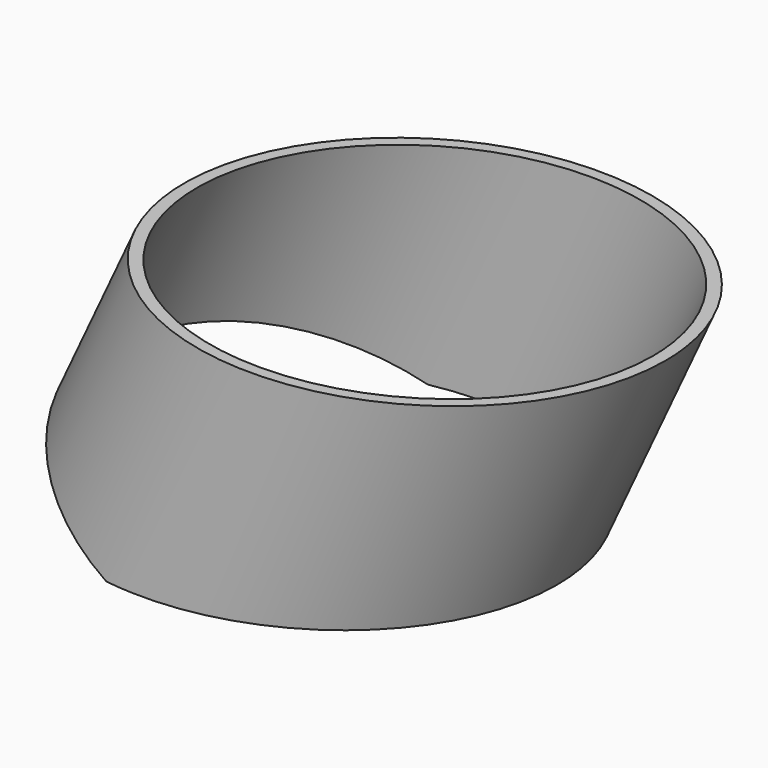
from build123d import *
from build123d import SkipClean  # not in build123d's __all__

# Parameters (mm, degrees)
F2_W     = 200
F2_H     = 100
F2_H_2   = 20
F3_DEPTH = 100
F2_W_2   = 75
F2_H_3   = 25
F6_DEPTH = 35
F8_W     = 96.0638802499
F8_H     = 5.2582259355
F9_DEPTH = 50


# Not quite as in the source:
# - ends of sketch curves that miss each other by under 0.0002 mm in the source are joined
# - a feature of the source that left no trace in its solid (it failed there, or was rolled back) is left out
# - a feature names something its author has since deleted; it is built from what else it names


with BuildPart() as f1:
    # F0 (on Front) → F1 (revolve)
    with BuildSketch(Plane.XZ):
        with BuildLine():
            add(Edge.make_bspline(
                [(45.9368361786, 26.8256458213), (91.5796084466, 124.7068868213), (26.32544778, 155.1354016666)],
                knots=[4.7123889804, 4.7123889804, 4.7123889804, 6.2831853072, 6.2831853072, 6.2831853072], degree=2, weights=[1, 0.7071067812, 1]))
            Line((26.32544778, 155.1354016666), (25.4802112565, 153.3227860925))
            add(Edge.make_bspline(
                [(44.1242206045, 27.6708823448), (88.921756349, 123.7395077707), (25.4802112565, 153.3227860925)],
                knots=[4.7123889804, 4.7123889804, 4.7123889804, 6.2831853072, 6.2831853072, 6.2831853072], degree=2, weights=[1, 0.7071067812, 1]))
            Line((44.1242206045, 27.6708823448), (45.9368361786, 26.8256458213))
        make_face()
    revolve(axis=Axis((-11.7101957767, 0, 73.5677008333), (-0.4226182617, 0, -0.906307787)))


with BuildPart() as f1b:
    # F0 (on Front) → F1, piece 2 (revolve)
    with BuildSketch(Plane.XZ):
        Polygon((0.1731735164, 31.6149234015), (-1.1862881642, 32.2488507941), (-15.9779273251, 0.5280782478), (-14.6184656445, -0.1058491448), align=None)
        with BuildLine():
            add(Edge.make_bspline(
                [(-22.1410875874, -12.6888615869), (-21.3247514691, -12.7218189818), (-20.5078685114, -12.7357143506)],
                knots=[0.3959818916, 0.3959818916, 0.3959818916, 0.4193237212, 0.4193237212, 0.4193237212], degree=2, weights=[1, 0.9999318956, 1]))
            Line((-20.5078685114, -12.7357143506), (-14.6184656445, -0.1058491448))
            Line((-14.6184656445, -0.1058491448), (-15.9779273251, 0.5280782478))
            Line((-15.9779273251, 0.5280782478), (-22.1410875874, -12.6888615869))
        make_face()
    revolve(axis=Axis((-11.7101957767, 0, 73.5677008333), (-0.4226182617, 0, -0.906307787)))


with BuildPart() as f3_tool:
    # F2 (on Front) → F3 (new body, symmetric)
    with BuildSketch(Plane.XZ):
        with Locations((-9.317324488, 115)):
            Rectangle(F2_W, F2_H)
        with Locations((0, -10)):
            Rectangle(F2_W, F2_H_2)
    extrude(amount=F3_DEPTH, both=True)


with BuildPart() as f1_1:
    add(f1.part, clean=False)

    # F3: cut by f3_tool
    add(f3_tool.part, mode=Mode.SUBTRACT)

    # F0 (on Front) → F7 (revolve, cut)
    with BuildSketch(Plane.XZ):
        with BuildLine():
            add(Edge.make_bspline(
                [(-84.5714851547, 87.682675512), (-114.9949652888, 22.4393118183), (-49.756636783, -7.9949639789)],
                knots=[4.7123889804, 4.7123889804, 4.7123889804, 6.2830198332, 6.2830198332, 6.2830198332], degree=2, weights=[1, 0.7071652827, 1]))
            Line((-49.756636783, -7.9949639789), (-49.7458393334, -8))
            Line((-49.7458393334, -8), (-49.735042102, -8.0050348317))
            add(Edge.make_bspline(
                [(-49.735042102, -8.0050348317), (15.5133557484, -38.4177185072), (45.9368361786, 26.8256458213)],
                knots=[0.0001654643, 0.0001654643, 0.0001654643, 1.5707963268, 1.5707963268, 1.5707963268], degree=2, weights=[1, 0.7071652792, 1]))
            Line((45.9368361786, 26.8256458213), (44.1242206045, 27.6708823448))
            add(Edge.make_bspline(
                [(-20.5078685114, -12.7357143506), (24.9219656119, -13.5084863764), (44.1242206045, 27.6708823448)],
                knots=[0.4193237212, 0.4193237212, 0.4193237212, 1.5707963268, 1.5707963268, 1.5707963268], degree=2, weights=[1, 0.8387916479, 1]))
            add(Edge.make_bspline(
                [(-22.1410875874, -12.6888615869), (-21.3247514691, -12.7218189818), (-20.5078685114, -12.7357143506)],
                knots=[0.3959818916, 0.3959818916, 0.3959818916, 0.4193237212, 0.4193237212, 0.4193237212], degree=2, weights=[1, 0.9999318956, 1]))
            add(Edge.make_bspline(
                [(-38.8967253804, -9.951843981), (-30.686098613, -12.3438795424), (-22.1410875874, -12.6888615869)],
                knots=[0.1528447244, 0.1528447244, 0.1528447244, 0.3959818916, 0.3959818916, 0.3959818916], degree=2, weights=[1, 0.9926196359, 1]))
            add(Edge.make_bspline(
                [(-48.9006028099, -6.1873844259), (-44.042789232, -8.4526200992), (-38.8967253804, -9.951843981)],
                knots=[0, 0, 0, 0.1528447244, 0.1528447244, 0.1528447244], degree=2, weights=[1, 0.9970812323, 1]))
            add(Edge.make_bspline(
                [(-48.9112500264, -6.1824184595), (-48.9059266265, -6.1849018895), (-48.9006028099, -6.1873844259)],
                knots=[6.2830174734, 6.2830174734, 6.2830174734, 6.2831853072, 6.2831853072, 6.2831853072], degree=2, weights=[1, 0.9999999965, 1]))
            add(Edge.make_bspline(
                [(-71.0817080874, 10.1325245471), (-61.6323129878, -0.2478899078), (-48.9112500264, -6.1824184595)],
                knots=[5.8872034156, 5.8872034156, 5.8872034156, 6.2830174734, 6.2830174734, 6.2830174734], degree=2, weights=[1, 0.9804802401, 1]))
            add(Edge.make_bspline(
                [(-72.1674123725, 11.3535265686), (-71.6316856587, 10.7366896891), (-71.0817080874, 10.1325245471)],
                knots=[5.863861586, 5.863861586, 5.863861586, 5.8872034156, 5.8872034156, 5.8872034156], degree=2, weights=[1, 0.9999318956, 1]))
            add(Edge.make_bspline(
                [(-82.7588695806, 86.8374389885), (-101.9611245733, 45.6580702673), (-72.1674123725, 11.3535265686)],
                knots=[4.7123889804, 4.7123889804, 4.7123889804, 5.863861586, 5.863861586, 5.863861586], degree=2, weights=[1, 0.8387916479, 1]))
            Line((-82.7588695806, 86.8374389885), (-84.5714851547, 87.682675512))
        make_face()
        with BuildLine():
            add(Edge.make_bspline(
                [(26.32544778, 155.1354016666), (-38.9287128867, 185.5639165119), (-84.5714851547, 87.682675512)],
                knots=[0, 0, 0, 1.5707963268, 1.5707963268, 1.5707963268], degree=2, weights=[1, 0.7071067812, 1]))
            Line((-84.5714851547, 87.682675512), (-82.7588695806, 86.8374389885))
            add(Edge.make_bspline(
                [(25.4802112565, 153.3227860925), (-37.9613338361, 182.9060644144), (-82.7588695806, 86.8374389885)],
                knots=[0, 0, 0, 1.5707963268, 1.5707963268, 1.5707963268], degree=2, weights=[1, 0.7071067812, 1]))
            Line((25.4802112565, 153.3227860925), (26.32544778, 155.1354016666))
        make_face()
    with SkipClean():  # cleaning this boolean's faces spoils the solid; the shape is the same uncleaned
        revolve(axis=Axis((-11.7101957767, 0, 73.5677008333), (-0.4226182617, 0, -0.906307787)), mode=Mode.SUBTRACT)


with BuildPart() as f1b_1:
    add(f1b.part, clean=False)

    # F3: cut by f3_tool
    add(f3_tool.part, mode=Mode.SUBTRACT)

    # F2 (on Front) → F6 (cut, symmetric)
    with BuildSketch(Plane.XZ):
        with Locations((-37.3268264836, 44.1149234015)):
            Rectangle(F2_W_2, F2_H_3)
    extrude(amount=F6_DEPTH, both=True, mode=Mode.SUBTRACT)

    # F8 (on Front) → F9 (cut, symmetric)
    with BuildSketch(Plane.XZ):
        with Locations((-19.0352806821, -1.4191129678)):
            Rectangle(F8_W, F8_H)
    extrude(amount=F9_DEPTH, both=True, mode=Mode.SUBTRACT)


solid = f1b_1.part
